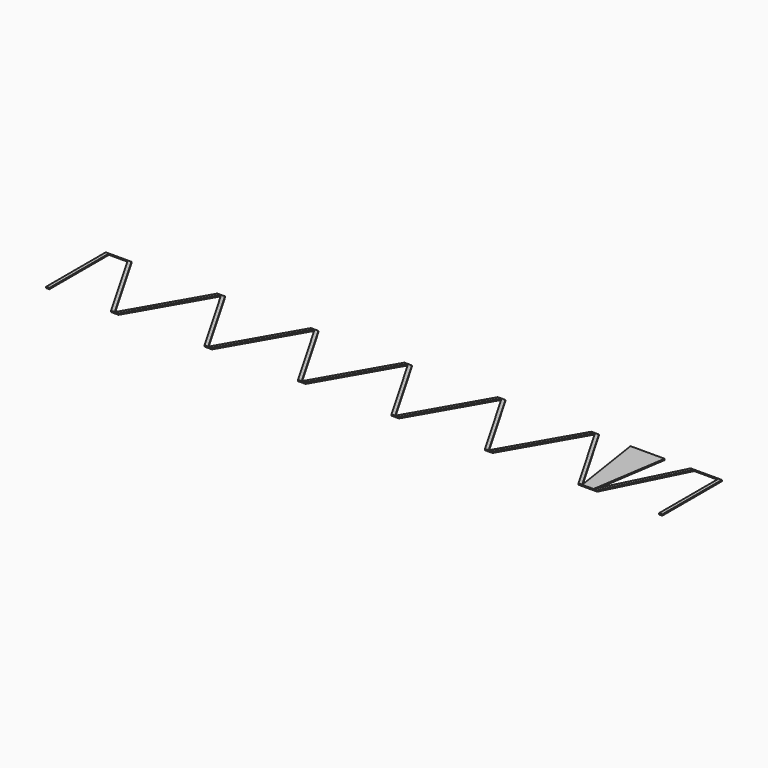
from build123d import *

# Parameters (mm, degrees)
F0_W     = 12.7
F0_H     = 0.254
F0_H_2   = 291.084
F0_W_2   = 9.525
F1_DEPTH = 4.7625


# Not quite as in the source:
# - a feature names something its author has since deleted; it is built from what else it names


with BuildPart() as f1:
    # F0 (on Top) → F1 (new body)
    with BuildSketch(Plane.XY):
        Polygon((-1095.375, 145.669), (-1168.4, 145.669), (-1168.4, 145.415), (-1095.2286143575, 145.415), align=None)
        with Locations((-1174.75, 145.542)):
            Rectangle(F0_W, F0_H)
        with Locations((-1174.75, -0.127)):
            Rectangle(F0_W, F0_H_2)
        with BuildLine():
            Line((1001.7125, 145.669), (935.0375, 145.669))
            Line((935.0375, 145.669), (935.0375, -145.669))
            Line((935.0375, -145.669), (971.4705200239, -145.669))
            Line((971.4705200239, -145.669), (1117.4725985353, 145.415))
            Line((1117.4725985353, 145.415), (1117.6, 145.669))
            Line((1117.6, 145.669), (1103.3919799761, 145.669))
            Line((1103.3919799761, 145.669), (957.9830261901, -144.232488632))
            ThreePointArc((957.9830261901, -144.232488632), (957.67894626, -144.3606444457), (957.5048911047, -144.080299445))
            Line((957.5048911047, -144.080299445), (1001.7125, 145.669))
        make_face()
        with BuildLine():
            Line((-1080.7168319418, 145.669), (-1095.375, 145.669))
            Line((-1095.375, 145.669), (-1095.2286143575, 145.415))
            Line((-1095.2286143575, 145.415), (-927.4706680582, -145.669))
            Line((-927.4706680582, -145.669), (-898.1543319418, -145.669))
            Line((-898.1543319418, -145.669), (-730.4700684279, 145.2871498423))
            ThreePointArc((-730.4700684279, 145.2871498423), (-730.25, 145.4143196918), (-730.0299315721, 145.2871498423))
            Line((-730.0299315721, 145.2871498423), (-562.3456680582, -145.669))
            Line((-562.3456680582, -145.669), (-533.0293319418, -145.669))
            Line((-533.0293319418, -145.669), (-365.3450684279, 145.2871498423))
            ThreePointArc((-365.3450684279, 145.2871498423), (-365.125, 145.4143196918), (-364.9049315721, 145.2871498423))
            Line((-364.9049315721, 145.2871498423), (-197.2206680582, -145.669))
            Line((-197.2206680582, -145.669), (-167.9043319418, -145.669))
            Line((-167.9043319418, -145.669), (-0.2200684279, 145.2871498423))
            ThreePointArc((-0.2200684279, 145.2871498423), (0, 145.4143196918), (0.2200684279, 145.2871498423))
            Line((0.2200684279, 145.2871498423), (167.9043319418, -145.669))
            Line((167.9043319418, -145.669), (197.2206680582, -145.669))
            Line((197.2206680582, -145.669), (364.9049315721, 145.2871498423))
            ThreePointArc((364.9049315721, 145.2871498423), (365.125, 145.4143196918), (365.3450684279, 145.2871498423))
            Line((365.3450684279, 145.2871498423), (533.0293319418, -145.669))
            Line((533.0293319418, -145.669), (562.3456680582, -145.669))
            Line((562.3456680582, -145.669), (730.0299315721, 145.2871498423))
            ThreePointArc((730.0299315721, 145.2871498423), (730.25, 145.4143196918), (730.4700684279, 145.2871498423))
            Line((730.4700684279, 145.2871498423), (898.1543319418, -145.669))
            Line((898.1543319418, -145.669), (935.0375, -145.669))
            Line((935.0375, -145.669), (935.0375, 145.669))
            Line((935.0375, 145.669), (868.3625, 145.669))
            Line((868.3625, 145.669), (912.6085893136, -144.3325111014))
            ThreePointArc((912.6085893136, -144.3325111014), (912.4415096754, -144.6105240597), (912.137426584, -144.4976511932))
            Line((912.137426584, -144.4976511932), (744.9081680582, 145.669))
            Line((744.9081680582, 145.669), (715.5918319418, 145.669))
            Line((715.5918319418, 145.669), (547.9075684279, -145.2871498423))
            ThreePointArc((547.9075684279, -145.2871498423), (547.6875, -145.4143196918), (547.4674315721, -145.2871498423))
            Line((547.4674315721, -145.2871498423), (379.7831680582, 145.669))
            Line((379.7831680582, 145.669), (350.4668319418, 145.669))
            Line((350.4668319418, 145.669), (182.7825684279, -145.2871498423))
            ThreePointArc((182.7825684279, -145.2871498423), (182.5625, -145.4143196918), (182.3424315721, -145.2871498423))
            Line((182.3424315721, -145.2871498423), (14.6581680582, 145.669))
            Line((14.6581680582, 145.669), (-14.6581680582, 145.669))
            Line((-14.6581680582, 145.669), (-182.3424315721, -145.2871498423))
            ThreePointArc((-182.3424315721, -145.2871498423), (-182.5625, -145.4143196918), (-182.7825684279, -145.2871498423))
            Line((-182.7825684279, -145.2871498423), (-350.4668319418, 145.669))
            Line((-350.4668319418, 145.669), (-379.7831680582, 145.669))
            Line((-379.7831680582, 145.669), (-547.4674315721, -145.2871498423))
            ThreePointArc((-547.4674315721, -145.2871498423), (-547.6875, -145.4143196918), (-547.9075684279, -145.2871498423))
            Line((-547.9075684279, -145.2871498423), (-715.5918319418, 145.669))
            Line((-715.5918319418, 145.669), (-744.9081680582, 145.669))
            Line((-744.9081680582, 145.669), (-912.5924315721, -145.2871498423))
            ThreePointArc((-912.5924315721, -145.2871498423), (-912.8125, -145.4143196918), (-913.0325684279, -145.2871498423))
            Line((-913.0325684279, -145.2871498423), (-1080.7168319418, 145.669))
        make_face()
        Polygon((1212.85, 145.415), (1212.85, -145.669), (1225.55, -145.669), (1225.55, 145.669), (1212.85, 145.669), align=None)
        Polygon((1117.6, 145.669), (1117.4725985353, 145.415), (1203.325, 145.415), (1203.325, 145.669), align=None)
        with Locations((1208.0875, 145.542)):
            Rectangle(F0_W_2, F0_H)
    extrude(amount=F1_DEPTH)


solid = f1.part
